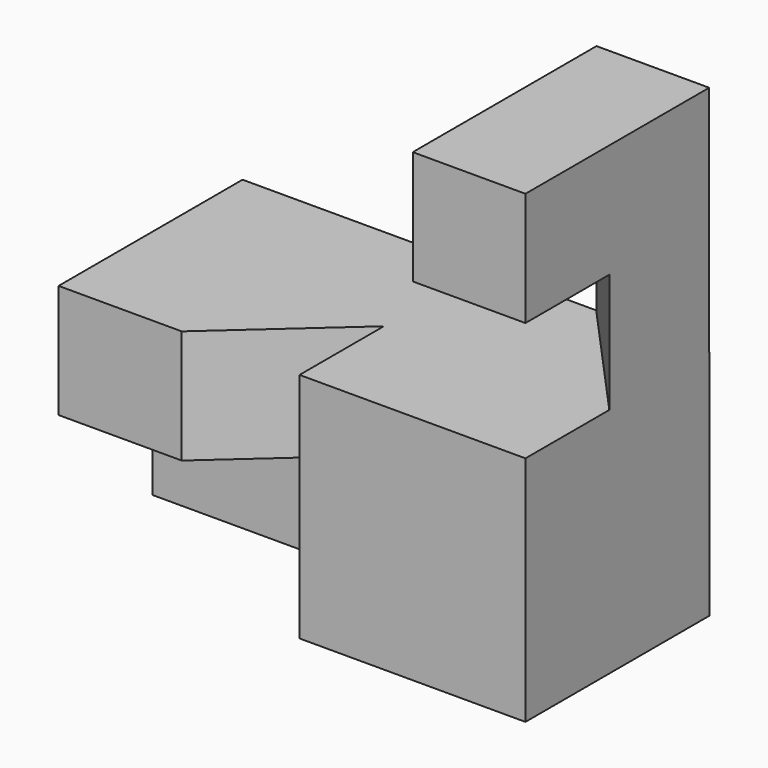
from build123d import *

# Parameters (mm, degrees)
F0_W      = 31.61
F0_H      = 15.57
F1_DEPTH  = 15.71
F2_W      = 7.63
F2_H      = 15.77
F3_DEPTH  = 15.55
F5_DEPTH  = 7.97
F7_DEPTH  = 25
F8_W      = 7.1303485631
F8_H      = 8.063195222
F9_DEPTH  = 25
F10_SIZE2 = 7.6
F10_SIZE  = 8.4


with BuildPart() as f1:
    # F0 (on Top) → F1 (new body)
    with BuildSketch(Plane.XY):
        with Locations((-0.5104932934, 0.6546514369)):
            Rectangle(F0_W, F0_H)
    extrude(amount=F1_DEPTH)

    # F2 (on face) → F3 (join)
    with BuildSketch(Plane.XZ.offset(7.1303485631)):
        with Locations((11.4795067066, 23.595)):
            Rectangle(F2_W, F2_H)
    extrude(amount=-F3_DEPTH)

    # F4 (on face) → F5 (cut)
    with BuildSketch(Plane.XZ.offset(7.1303485631)):
        Polygon((-0.4054932934, 0), (-0.4054932934, 8.01), (-8.0654932934, 8.01), (-16.3154932934, 8.01), (-16.3154932934, 0), align=None)
    extrude(amount=-F5_DEPTH, mode=Mode.SUBTRACT)

    # F6 (on face) → F7 (cut)
    with BuildSketch(Plane.XY.offset(15.71)):
        Polygon((0, 0), (-7.9760523513, -7.1303485631), (0, -7.1303485631), align=None)
    extrude(amount=-F7_DEPTH, mode=Mode.SUBTRACT)

    # F8 (on face) → F9 (cut)
    with BuildSketch(Plane.YZ.offset(15.2945067066)):
        with Locations((-3.5651742816, 19.741597611)):
            Rectangle(F8_W, F8_H)
    extrude(amount=-F9_DEPTH, mode=Mode.SUBTRACT)

    # F10
    f10_edges = [f1.edges().sort_by_distance(p)[0] for p in [
        (7.664507, 0, 19.741598),
    ]]
    f10_side = f1.faces().sort_by_distance((7.664507, 1.933934, 24.775126))[0]
    chamfer(f10_edges, length=F10_SIZE, length2=F10_SIZE2, reference=f10_side)


solid = f1.part
